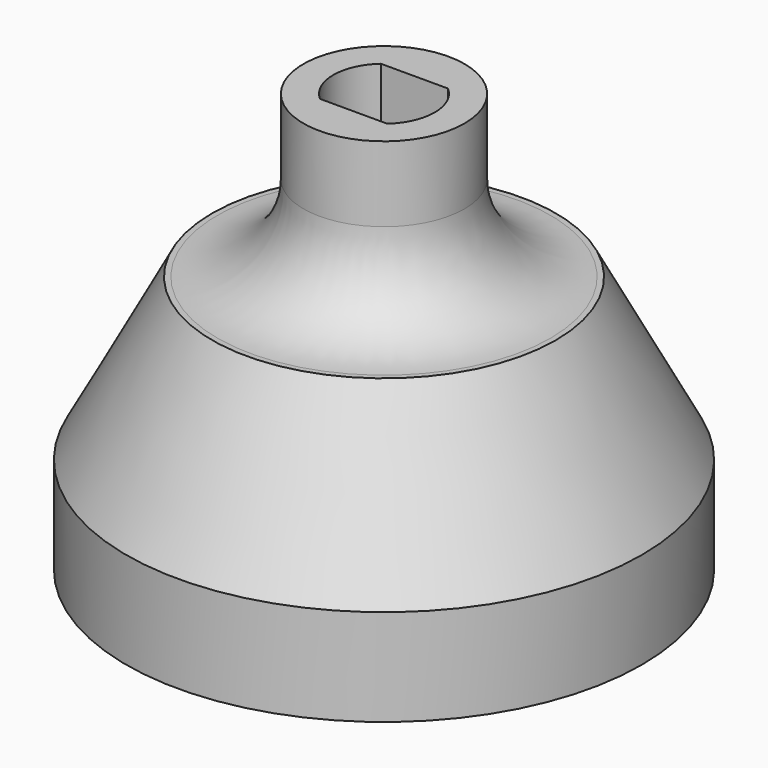
from build123d import *

# Parameters (mm, degrees)
F0_R          = 4.7625
F1_DEPTH      = 9.525
F1_DEPTH_BACK = 6.35
F3_DEPTH      = 9.526
F4_R          = 15.24
F5_DEPTH      = 15.24
F6_R          = 2.413
F7_DEPTH      = 13.97
F8_SIZE2      = 9.525
F8_SIZE       = 5.08
F9_R          = 5.08


with BuildPart() as f1:
    # F0 (on Top) → F1 (new body, two sides)
    with BuildSketch(Plane.XY) as f1_sk:
        Circle(F0_R)
    extrude(amount=F1_DEPTH)
    extrude(f1_sk.sketch, amount=-F1_DEPTH_BACK)

    # F2 (on Top) → F3 (cut, through all)
    with BuildSketch(Plane.XY):
        with BuildLine():
            ThreePointArc((1.9843134833, -2.25), (2.7343134833, -1.2343134833), (3, 0))
            ThreePointArc((3, 0), (2.7343134833, 1.2343134833), (1.9843134833, 2.25))
            Line((1.9843134833, 2.25), (-1.9843134833, 2.25))
            ThreePointArc((-1.9843134833, 2.25), (-3, 0), (-1.9843134833, -2.25))
            Line((-1.9843134833, -2.25), (1.9843134833, -2.25))
        make_face()
    extrude(amount=F3_DEPTH, mode=Mode.SUBTRACT)

    # F4 (on Top) → F5 (join)
    with BuildSketch(Plane.XY):
        Circle(F4_R)
    extrude(amount=-F5_DEPTH)

    # F6 (on face) → F7 (cut)
    with BuildSketch(Plane(origin=(0, 0, -15.24), x_dir=(1, 0, 0), z_dir=(0, 0, -1))):
        with Locations((1.0674559099, -7.8653953575)):
            Circle(F6_R)
        with Locations((6.2779042355, 4.8571416142)):
            Circle(F6_R)
        with Locations((-7.3453601454, 3.0082537434)):
            Circle(F6_R)
    extrude(amount=-F7_DEPTH, mode=Mode.SUBTRACT)

    # F8
    f8_edges = [f1.edges().sort_by_distance(p)[0] for p in [
        (-15.24, 0, 0),
    ]]
    f8_side = f1.faces().sort_by_distance((-14.808948, 0, 0))[0]
    chamfer(f8_edges, length=F8_SIZE, length2=F8_SIZE2, reference=f8_side)

    # F9
    f9_edges = [f1.edges().sort_by_distance(p)[0] for p in [
        (-4.7625, 0, 0),
    ]]
    fillet(f9_edges, radius=F9_R)


solid = f1.part
